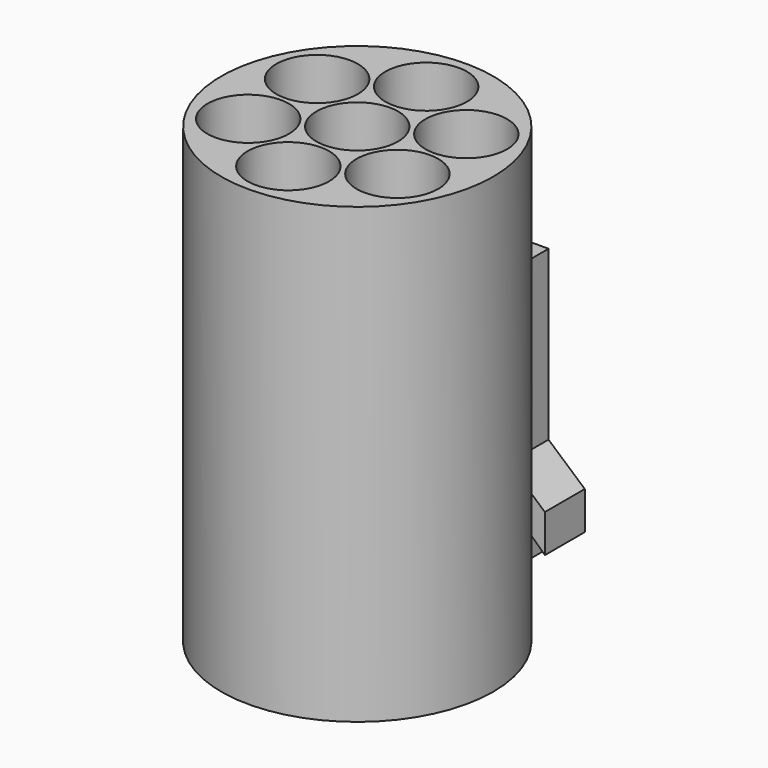
from build123d import *

# Parameters (mm, degrees)
F2_R      = 1.5
F3_DEPTH  = 5
F9_DEPTH  = 0.55
F1_R      = 0.45
F10_DEPTH = 5.001


with BuildPart() as f3:
    # F2 (on Top) → F3 (new body)
    with BuildSketch(Plane.XY):
        Circle(F2_R)
    extrude(amount=F3_DEPTH)

    # F8 (on face) → F9 (join)
    with BuildSketch(Plane(origin=(0, 1.15, 0), x_dir=(-1, 0, 0), z_dir=(0, 1, 0))):
        Polygon((0.9573300485, 2.7517464478), (0.9876711119, 3.0308461282), (0.7235942503, 2.8000105567), (0.7235942503, 2.5290050786), align=None)
        Polygon((0.7235942503, 2.5290050786), (0.7235942503, 2.8000105567), (0.3857031334, 2.5046522711), (0.3857031334, 2.2070076328), align=None)
        Polygon((0.3857031334, 2.5046522711), (0.7235942503, 2.8000105567), (0.7235942503, 3.3656487685), (0.3857031334, 3.3656487685), align=None)
        Polygon((0.7235942503, 0.4582579713), (0.7235942503, 2.5290050786), (0.3857031334, 2.2070076328), (0.3857031334, 0.4582579713), align=None)
        Polygon((0.3857031334, 2.2070076328), (0.3857031334, 2.5046522711), (0.1338190596, 2.2844746918), (0.1338190596, 1.966971644), align=None)
        Polygon((0.1338190596, 1.966971644), (0.1338190596, 2.2844746918), (-0.2040720574, 1.9891164063), (-0.2040720574, 1.6449741982), align=None)
        Polygon((-0.2040720574, 1.9891164063), (0.1338190596, 2.2844746918), (0.1338190596, 3.3656487685), (-0.2040720574, 3.3656487685), align=None)
        Polygon((0.1338190596, 0.4582579713), (0.1338190596, 1.966971644), (-0.2040720574, 1.6449741982), (-0.2040720574, 0.4582579713), align=None)
        Polygon((-0.2040720574, 1.6449741982), (-0.2040720574, 1.9891164063), (-0.4116180899, 1.8076957141), (-0.4116180899, 1.4471906846), align=None)
        Polygon((-0.4116180899, 1.4471906846), (-0.4116180899, 1.8076957141), (-0.7495092068, 1.5123374285), (-0.7495092068, 1.1251932388), align=None)
        Polygon((-0.7495092068, 1.5123374285), (-0.4116180899, 1.8076957141), (-0.4116180899, 3.3656487685), (-0.7495092068, 3.3656487685), align=None)
        Polygon((-0.4116180899, 0.4582579713), (-0.4116180899, 1.4471906846), (-0.7495092068, 1.1251932388), (-0.7495092068, 0.4582579713), align=None)
        Polygon((-0.7495092068, 1.1251932388), (-0.7495092068, 1.5123374285), (-1.1491243131, 1.1630248046), (-1.1491243131, 0.7443751674), align=None)
    extrude(amount=F9_DEPTH)

    # F1 (on Top) → F10 (cut, through all)
    with BuildSketch(Plane.XY):
        Circle(F1_R)
        with Locations((0, 0.95)):
            Circle(F1_R)
        with Locations((0.8227241336, 0.475)):
            Circle(F1_R)
        with Locations((0.8227241336, -0.475)):
            Circle(F1_R)
        with Locations((0, -0.95)):
            Circle(F1_R)
        with Locations((-0.8227241336, -0.475)):
            Circle(F1_R)
        with Locations((-0.8227241336, 0.475)):
            Circle(F1_R)
    extrude(amount=F10_DEPTH, mode=Mode.SUBTRACT)


solid = f3.part
